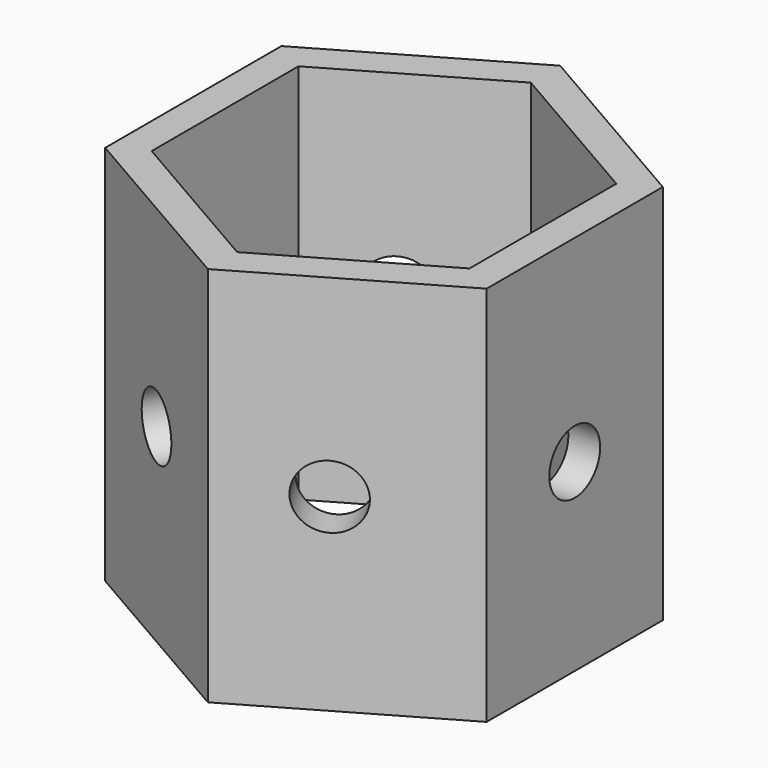
from build123d import *

# Parameters (mm, degrees)
F1_DEPTH = 6
F2_R     = 0.5
F3_DEPTH = 10
F4_R     = 0.5
F5_DEPTH = 10
F6_R     = 0.5
F7_DEPTH = 10


with BuildPart() as f1:
    # F0 (on Top) → F1 (new body)
    with BuildSketch(Plane.XY):
        Polygon((-3, 1.7320508076), (-3, -1.7320508076), (0, -3.4641016151), (3, -1.7320508076), (3, 1.7320508076), (0, 3.4641016151), align=None)
        Polygon((0, -2.8867513459), (-2.5, -1.443375673), (-2.5, 1.443375673), (0, 2.8867513459), (2.5, 1.443375673), (2.5, -1.443375673), align=None, mode=Mode.SUBTRACT)
    extrude(amount=F1_DEPTH)

    # F2 (on face) → F3 (cut)
    with BuildSketch(Plane.YZ.offset(3)):
        with Locations((0, 2.8977813589)):
            Circle(F2_R)
    extrude(amount=-F3_DEPTH, mode=Mode.SUBTRACT)

    # F4 (on face) → F5 (cut)
    with BuildSketch(Plane(origin=(1.5, 2.5980762114, 0), x_dir=(-0.8660254038, 0.5, 0), z_dir=(0.5, 0.8660254038, 0))):
        with Locations((0, 2.9807699823)):
            Circle(F4_R)
    extrude(amount=-F5_DEPTH, mode=Mode.SUBTRACT)

    # F6 (on face) → F7 (cut)
    with BuildSketch(Plane(origin=(-1.5, 2.5980762114, 0), x_dir=(-0.8660254038, -0.5, 0), z_dir=(-0.5, 0.8660254038, 0))):
        with Locations((0.2181102464, 2.9651848599)):
            Circle(F6_R)
    extrude(amount=-F7_DEPTH, mode=Mode.SUBTRACT)


solid = f1.part
